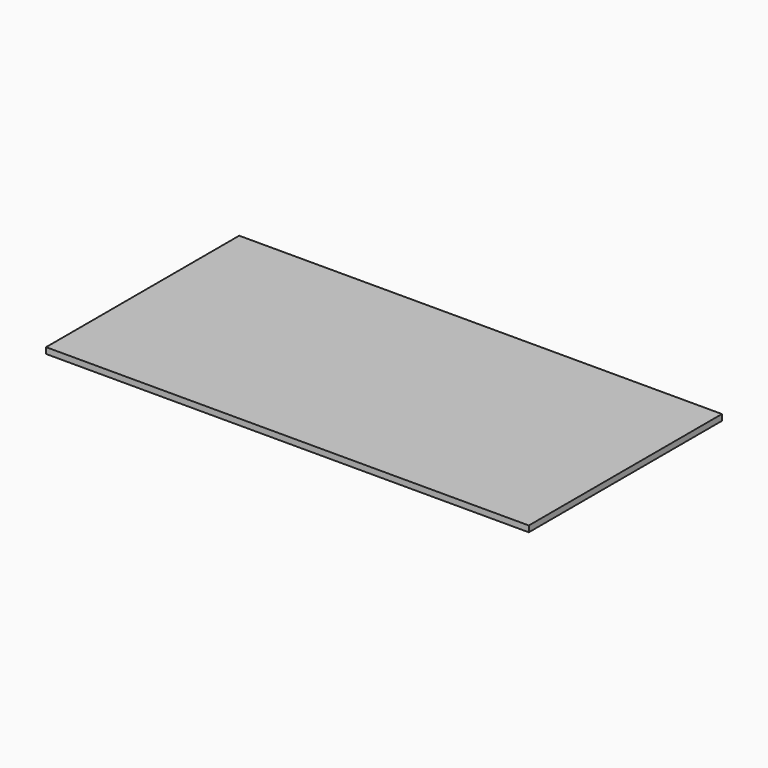
from build123d import *

# Parameters (mm, degrees)
F0_W     = 1016
F0_H     = 508
F1_DEPTH = 6.35


# Not quite as in the source:
# - the program builds the solid bodies; features that only make, move or delete a surface that nothing else refers to are left out


with BuildPart() as f1:
    # F0 (on Top) → F1 (new body, symmetric)
    with BuildSketch(Plane.XY):
        Rectangle(F0_W, F0_H)
    extrude(amount=F1_DEPTH, both=True)


solid = f1.part
